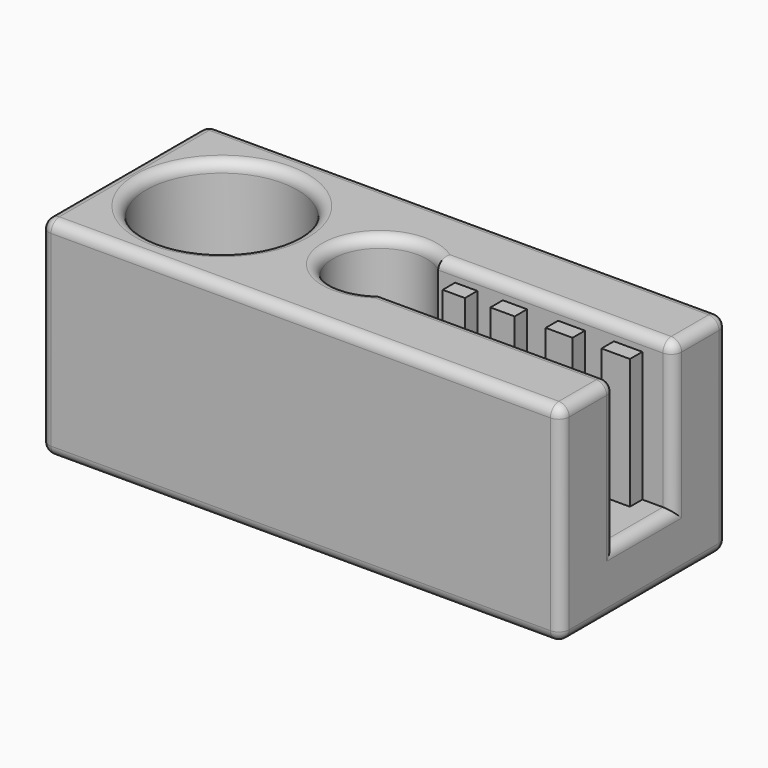
from build123d import *

# Parameters (mm, degrees)
F0_W           = 25.4
F0_H           = 10.16
F1_DEPTH       = 10.16
F2_R           = 3.6858409811
F3_DEPTH       = 6.35
F4_R           = 2.286
F5_DEPTH       = 10.161
F6_R           = 2.032
F7_DEPTH       = 3.811
F8_W           = 1.78028786
F8_H           = 7.1321626426
F9_DEPTH       = 12.7
F10_W          = 1.08565134
F10_H          = 0.7570284122
F10_W_2        = 1.1861119419
F10_W_3        = 1.3122945093
F10_W_4        = 1.3880031183
F11_DEPTH      = 6.35
F12_T1_DEPTH   = 9.144
F12_T3_DEPTH   = 2.28371214
F12_T5_DEPTH   = 6.6241626426
F12_T7_DEPTH   = 3.5605757201
F12_T9_DEPTH   = 2.28371214
F12_T11_DEPTH  = 9.144
F12_T13_DEPTH  = 24.384
F12_T15_DEPTH  = 12.2405523365
F12_S19_W      = 0.508
F12_S19_H      = 0.508
F12_T20_DEPTH  = 0.508
F12_S25_W      = 0.508
F12_S25_H      = 0.508
F12_T26_DEPTH  = 0.508
F12_S31_W      = 0.508
F12_S31_H      = 0.508
F12_T32_DEPTH  = 0.508
F12_S37_W      = 0.508
F12_S37_H      = 0.508
F12_T38_DEPTH  = 0.508
F12_S43_W      = 0.508
F12_S43_H      = 0.508
F12_T44_DEPTH  = 0.508
F12_S49_W      = 0.508
F12_S49_H      = 0.508
F12_T50_DEPTH  = 0.508
F12_S55_W      = 0.508
F12_S55_H      = 0.508
F12_T56_DEPTH  = 0.508
F12_S61_W      = 0.508
F12_S61_H      = 0.508
F12_T62_DEPTH  = 0.508
F12_S67_W      = 0.508
F12_S67_H      = 0.508
F12_T68_DEPTH  = 0.508
F12_S73_W      = 0.508
F12_S73_H      = 0.508
F12_T74_DEPTH  = 0.508
F12_T80_ANGLE  = 321.5743152005
F12_T86_ANGLE  = 82.9839978372
F12_T93_ANGLE  = 82.9839978372
F12_T99_ANGLE  = 82.9839978372
F12_T105_ANGLE = 82.9839978372
F12_T111_ANGLE = 82.9839978372
F12_T117_ANGLE = 82.9839978372
F12_T129_DEPTH = 7.8941626426
F12_T133_DEPTH = 4.8305757201
F12_T140_DEPTH = 4.8305757201
F12_T144_DEPTH = 7.8941626426


# Not quite as in the source:
# - a fillet or chamfer that OpenCascade refuses, or shapes differently, is made with other operations: its cross-section is extruded or revolved along the edge and cut away or added


with BuildPart() as f1:
    # F0 (on Front) → F1 (new body)
    with BuildSketch(Plane.XZ):
        with Locations((0.2125576138, 0.3190716813)):
            Rectangle(F0_W, F0_H)
    extrude(amount=F1_DEPTH)

    # F2 (on face) → F3 (cut)
    with BuildSketch(Plane.XY.offset(5.3990716813)):
        with Locations((-7.7062794007, -5.08)):
            Circle(F2_R)
    extrude(amount=-F3_DEPTH, mode=Mode.SUBTRACT)

    # F4 (on face) → F5 (cut, through all)
    with BuildSketch(Plane.XY.offset(5.3990716813)):
        with Locations((0, -5.08)):
            Circle(F4_R)
    extrude(amount=-F5_DEPTH, mode=Mode.SUBTRACT)

    # F6 (on face) → F7 (cut, through all)
    with BuildSketch(Plane.XY.offset(-0.9509283187)):
        with Locations((-7.7062794007, -5.08)):
            Circle(F6_R)
    extrude(amount=-F7_DEPTH, mode=Mode.SUBTRACT)

    # F8 (on face) → F9 (cut)
    with BuildSketch(Plane.YZ.offset(12.9125576138)):
        with Locations((-5.97014393, 1.83299036)):
            Rectangle(F8_W, F8_H)
        with Locations((-4.18985607, 1.83299036)):
            Rectangle(F8_W, F8_H)
    extrude(amount=-F9_DEPTH, mode=Mode.SUBTRACT)

    # F10 (on face) → F11 (join)
    with BuildSketch(Plane.XY.offset(-1.7330909614)):
        with Locations((2.8024074854, -3.6782263461)):
            Rectangle(F10_W, F10_H)
        with Locations((5.1806154661, -3.6782263461)):
            Rectangle(F10_W_2, F10_H)
        with Locations((7.9440039117, -3.6782263461)):
            Rectangle(F10_W_3, F10_H)
        with Locations((10.7073918916, -3.6782263461)):
            Rectangle(F10_W_4, F10_H)
        with Locations((2.8024074854, -6.4817736539)):
            Rectangle(F10_W, F10_H)
        with Locations((5.1806154661, -6.4817736539)):
            Rectangle(F10_W_2, F10_H)
        with Locations((7.9440039117, -6.4817736539)):
            Rectangle(F10_W_3, F10_H)
        with Locations((10.7073918916, -6.4817736539)):
            Rectangle(F10_W_4, F10_H)
    extrude(amount=F11_DEPTH)

    # F12: fillet of radius 0.508 on 25 edges, made by hand

    # F12_s2 → F12_t1 (cut)
    with BuildSketch(Plane.XY.offset(-4.2529283187)):
        with BuildLine():
            ThreePointArc((12.4045576138, 0), (12.7637678587, -0.1487897552), (12.9125576138, -0.508))
            Line((12.9125576138, -0.508), (12.9125576138, 0))
            Line((12.9125576138, 0), (12.4045576138, 0))
        make_face()
        with BuildLine():
            ThreePointArc((12.4045576138, -10.16), (12.7637678587, -10.0112102448), (12.9125576138, -9.652))
            Line((12.9125576138, -9.652), (12.9125576138, -10.16))
            Line((12.9125576138, -10.16), (12.4045576138, -10.16))
        make_face()
        with BuildLine():
            ThreePointArc((-11.9794423862, 0), (-12.338652631, -0.1487897552), (-12.4874423862, -0.508))
            Line((-12.4874423862, -0.508), (-12.4874423862, 0))
            Line((-12.4874423862, 0), (-11.9794423862, 0))
        make_face()
        with BuildLine():
            ThreePointArc((-12.4874423862, -9.652), (-12.338652631, -10.0112102448), (-11.9794423862, -10.16))
            Line((-11.9794423862, -10.16), (-12.4874423862, -10.16))
            Line((-12.4874423862, -10.16), (-12.4874423862, -9.652))
        make_face()
    extrude(amount=F12_T1_DEPTH, mode=Mode.SUBTRACT)

    # F12_s4 → F12_t3 (cut)
    with BuildSketch(Plane.XZ.offset(0.508)):
        with BuildLine():
            ThreePointArc((12.4045576138, 5.3990716813), (12.7637678587, 5.2502819261), (12.9125576138, 4.8910716813))
            Line((12.9125576138, 4.8910716813), (12.9125576138, 5.3990716813))
            Line((12.9125576138, 5.3990716813), (12.4045576138, 5.3990716813))
        make_face()
    extrude(amount=F12_T3_DEPTH, mode=Mode.SUBTRACT)

    # F12_s6 → F12_t5 (cut)
    with BuildSketch(Plane.XY.offset(-1.7330909614)):
        with BuildLine():
            ThreePointArc((12.9125576138, -2.79171214), (12.7637678587, -3.1509223848), (12.4045576138, -3.29971214))
            Line((12.4045576138, -3.29971214), (12.9125576138, -3.29971214))
            Line((12.9125576138, -3.29971214), (12.9125576138, -2.79171214))
        make_face()
        with BuildLine():
            ThreePointArc((12.9125576138, -7.36828786), (12.7637678587, -7.0090776152), (12.4045576138, -6.86028786))
            Line((12.4045576138, -6.86028786), (12.9125576138, -6.86028786))
            Line((12.9125576138, -6.86028786), (12.9125576138, -7.36828786))
        make_face()
    extrude(amount=F12_T5_DEPTH, mode=Mode.SUBTRACT)

    # F12_s8 → F12_t7 (cut)
    with BuildSketch(Plane.XZ.offset(3.29971214)):
        with BuildLine():
            ThreePointArc((12.9125576138, -2.2410909614), (12.7637678587, -1.8818807165), (12.4045576138, -1.7330909614))
            Line((12.4045576138, -1.7330909614), (12.9125576138, -1.7330909614))
            Line((12.9125576138, -1.7330909614), (12.9125576138, -2.2410909614))
        make_face()
    extrude(amount=F12_T7_DEPTH, mode=Mode.SUBTRACT)

    # F12_s10 → F12_t9 (cut)
    with BuildSketch(Plane.XZ.offset(7.36828786)):
        with BuildLine():
            ThreePointArc((12.4045576138, 5.3990716813), (12.7637678587, 5.2502819261), (12.9125576138, 4.8910716813))
            Line((12.9125576138, 4.8910716813), (12.9125576138, 5.3990716813))
            Line((12.9125576138, 5.3990716813), (12.4045576138, 5.3990716813))
        make_face()
    extrude(amount=F12_T9_DEPTH, mode=Mode.SUBTRACT)

    # F12_s12 → F12_t11 (cut)
    with BuildSketch(Plane.XZ.offset(0.508)):
        with BuildLine():
            ThreePointArc((12.9125576138, -4.2529283187), (12.7637678587, -4.6121385636), (12.4045576138, -4.7609283187))
            Line((12.4045576138, -4.7609283187), (12.9125576138, -4.7609283187))
            Line((12.9125576138, -4.7609283187), (12.9125576138, -4.2529283187))
        make_face()
        with BuildLine():
            ThreePointArc((-12.4874423862, -4.2529283187), (-12.338652631, -4.6121385636), (-11.9794423862, -4.7609283187))
            Line((-11.9794423862, -4.7609283187), (-12.4874423862, -4.7609283187))
            Line((-12.4874423862, -4.7609283187), (-12.4874423862, -4.2529283187))
        make_face()
        with BuildLine():
            ThreePointArc((-11.9794423862, 5.3990716813), (-12.338652631, 5.2502819261), (-12.4874423862, 4.8910716813))
            Line((-12.4874423862, 4.8910716813), (-12.4874423862, 5.3990716813))
            Line((-12.4874423862, 5.3990716813), (-11.9794423862, 5.3990716813))
        make_face()
    extrude(amount=F12_T11_DEPTH, mode=Mode.SUBTRACT)

    # F12_s14 → F12_t13 (cut)
    with BuildSketch(Plane.YZ.offset(-11.9794423862)):
        with BuildLine():
            ThreePointArc((-0.508, 5.3990716813), (-0.1487897552, 5.2502819261), (0, 4.8910716813))
            Line((0, 4.8910716813), (0, 5.3990716813))
            Line((0, 5.3990716813), (-0.508, 5.3990716813))
        make_face()
        with BuildLine():
            ThreePointArc((-9.652, 5.3990716813), (-10.0112102448, 5.2502819261), (-10.16, 4.8910716813))
            Line((-10.16, 4.8910716813), (-10.16, 5.3990716813))
            Line((-10.16, 5.3990716813), (-9.652, 5.3990716813))
        make_face()
        with BuildLine():
            ThreePointArc((0, -4.2529283187), (-0.1487897552, -4.6121385636), (-0.508, -4.7609283187))
            Line((-0.508, -4.7609283187), (0, -4.7609283187))
            Line((0, -4.7609283187), (0, -4.2529283187))
        make_face()
        with BuildLine():
            ThreePointArc((-10.16, -4.2529283187), (-10.0112102448, -4.6121385636), (-9.652, -4.7609283187))
            Line((-9.652, -4.7609283187), (-10.16, -4.7609283187))
            Line((-10.16, -4.7609283187), (-10.16, -4.2529283187))
        make_face()
    extrude(amount=F12_T13_DEPTH, mode=Mode.SUBTRACT)

    # F12_s16 → F12_t15 (cut)
    with BuildSketch(Plane.YZ.offset(0.1640052773)):
        with BuildLine():
            ThreePointArc((-7.36828786, 5.3990716813), (-7.0090776152, 5.2502819261), (-6.86028786, 4.8910716813))
            Line((-6.86028786, 4.8910716813), (-6.86028786, 5.3990716813))
            Line((-6.86028786, 5.3990716813), (-7.36828786, 5.3990716813))
        make_face()
        with BuildLine():
            ThreePointArc((-2.79171214, 5.3990716813), (-3.1509223848, 5.2502819261), (-3.29971214, 4.8910716813))
            Line((-3.29971214, 4.8910716813), (-3.29971214, 5.3990716813))
            Line((-3.29971214, 5.3990716813), (-2.79171214, 5.3990716813))
        make_face()
    extrude(amount=F12_T15_DEPTH, mode=Mode.SUBTRACT)


with BuildPart() as f12_tool18:
    # F12_s19 → F12_t20 (new body)
    with BuildSketch(Plane.XZ.offset(0.508)):
        with Locations((12.6585576138, -4.5069283187)):
            Rectangle(F12_S19_W, F12_S19_H)
    extrude(amount=-F12_T20_DEPTH)

    # F12_s21 → F12_t22 (revolve, cut)
    with BuildSketch(Plane(origin=(12.4045576138, -0.508, -4.2529283187), x_dir=(-0.7071067812, 0, 0.7071067812), z_dir=(-0.7071067812, 0, -0.7071067812))):
        with BuildLine():
            ThreePointArc((0, -0.508), (0.508, 0), (0, 0.508))
            Line((0, 0.508), (0, -0.508))
        make_face()
    revolve(axis=Axis((12.4045576138, -0.508, -4.2529283187), (0, 1, 0)), mode=Mode.SUBTRACT)


with BuildPart() as f1_1:
    add(f1.part)

    # F12_t17: cut F12_tool18
    add(f12_tool18.part, mode=Mode.SUBTRACT)


with BuildPart() as f12_tool24:
    # F12_s25 → F12_t26 (new body)
    with BuildSketch(Plane.XY.offset(4.8910716813)):
        with Locations((12.6585576138, -0.254)):
            Rectangle(F12_S25_W, F12_S25_H)
    extrude(amount=F12_T26_DEPTH)

    # F12_s27 → F12_t28 (revolve, cut)
    with BuildSketch(Plane(origin=(12.4045576138, -0.508, 4.8910716813), x_dir=(-0.7071067812, -0.7071067812, 0), z_dir=(-0.7071067812, 0.7071067812, 0))):
        with BuildLine():
            ThreePointArc((0, -0.508), (0.508, 0), (0, 0.508))
            Line((0, 0.508), (0, -0.508))
        make_face()
    revolve(axis=Axis((12.4045576138, -0.508, 4.8910716813), (0, 0, 1)), mode=Mode.SUBTRACT)


with BuildPart() as f1_2:
    add(f1_1.part)

    # F12_t23: cut F12_tool24
    add(f12_tool24.part, mode=Mode.SUBTRACT)


with BuildPart() as f12_tool30:
    # F12_s31 → F12_t32 (new body)
    with BuildSketch(Plane.XY.offset(4.8910716813)):
        with Locations((12.6585576138, -3.04571214)):
            Rectangle(F12_S31_W, F12_S31_H)
    extrude(amount=F12_T32_DEPTH)

    # F12_s33 → F12_t34 (revolve, cut)
    with BuildSketch(Plane(origin=(12.4045576138, -2.79171214, 4.8910716813), x_dir=(-0.7071067812, 0.7071067812, 0), z_dir=(0.7071067812, 0.7071067812, 0))):
        with BuildLine():
            ThreePointArc((0, -0.508), (0.508, 0), (0, 0.508))
            Line((0, 0.508), (0, -0.508))
        make_face()
    revolve(axis=Axis((12.4045576138, -2.79171214, 4.8910716813), (0, 0, 1)), mode=Mode.SUBTRACT)


with BuildPart() as f1_3:
    add(f1_2.part)

    # F12_t29: cut F12_tool30
    add(f12_tool30.part, mode=Mode.SUBTRACT)


with BuildPart() as f12_tool36:
    # F12_s37 → F12_t38 (new body)
    with BuildSketch(Plane.XY.offset(4.8910716813)):
        with Locations((12.6585576138, -7.11428786)):
            Rectangle(F12_S37_W, F12_S37_H)
    extrude(amount=F12_T38_DEPTH)

    # F12_s39 → F12_t40 (revolve, cut)
    with BuildSketch(Plane(origin=(12.4045576138, -7.36828786, 4.8910716813), x_dir=(-0.7071067812, -0.7071067812, 0), z_dir=(-0.7071067812, 0.7071067812, 0))):
        with BuildLine():
            ThreePointArc((0, -0.508), (0.508, 0), (0, 0.508))
            Line((0, 0.508), (0, -0.508))
        make_face()
    revolve(axis=Axis((12.4045576138, -7.36828786, 4.8910716813), (0, 0, 1)), mode=Mode.SUBTRACT)


with BuildPart() as f1_4:
    add(f1_3.part)

    # F12_t35: cut F12_tool36
    add(f12_tool36.part, mode=Mode.SUBTRACT)


with BuildPart() as f12_tool42:
    # F12_s43 → F12_t44 (new body)
    with BuildSketch(Plane.XY.offset(4.8910716813)):
        with Locations((12.6585576138, -9.906)):
            Rectangle(F12_S43_W, F12_S43_H)
    extrude(amount=F12_T44_DEPTH)

    # F12_s45 → F12_t46 (revolve, cut)
    with BuildSketch(Plane(origin=(12.4045576138, -9.652, 4.8910716813), x_dir=(-0.7071067812, 0.7071067812, 0), z_dir=(0.7071067812, 0.7071067812, 0))):
        with BuildLine():
            ThreePointArc((0, -0.508), (0.508, 0), (0, 0.508))
            Line((0, 0.508), (0, -0.508))
        make_face()
    revolve(axis=Axis((12.4045576138, -9.652, 4.8910716813), (0, 0, 1)), mode=Mode.SUBTRACT)


with BuildPart() as f1_5:
    add(f1_4.part)

    # F12_t41: cut F12_tool42
    add(f12_tool42.part, mode=Mode.SUBTRACT)


with BuildPart() as f12_tool48:
    # F12_s49 → F12_t50 (new body)
    with BuildSketch(Plane.XY.offset(-4.2529283187)):
        with Locations((12.6585576138, -9.906)):
            Rectangle(F12_S49_W, F12_S49_H)
    extrude(amount=-F12_T50_DEPTH)

    # F12_s51 → F12_t52 (revolve, cut)
    with BuildSketch(Plane(origin=(12.4045576138, -9.652, -4.2529283187), x_dir=(-0.7071067812, 0.7071067812, 0), z_dir=(-0.7071067812, -0.7071067812, 0))):
        with BuildLine():
            ThreePointArc((0, -0.508), (0.508, 0), (0, 0.508))
            Line((0, 0.508), (0, -0.508))
        make_face()
    revolve(axis=Axis((12.4045576138, -9.652, -4.2529283187), (0, 0, -1)), mode=Mode.SUBTRACT)


with BuildPart() as f1_6:
    add(f1_5.part)

    # F12_t47: cut F12_tool48
    add(f12_tool48.part, mode=Mode.SUBTRACT)


with BuildPart() as f12_tool54:
    # F12_s55 → F12_t56 (new body)
    with BuildSketch(Plane.XY.offset(4.8910716813)):
        with Locations((-12.2334423862, -0.254)):
            Rectangle(F12_S55_W, F12_S55_H)
    extrude(amount=F12_T56_DEPTH)

    # F12_s57 → F12_t58 (revolve, cut)
    with BuildSketch(Plane(origin=(-11.9794423862, -0.508, 4.8910716813), x_dir=(0.7071067812, -0.7071067812, 0), z_dir=(-0.7071067812, -0.7071067812, 0))):
        with BuildLine():
            ThreePointArc((0, -0.508), (0.508, 0), (0, 0.508))
            Line((0, 0.508), (0, -0.508))
        make_face()
    revolve(axis=Axis((-11.9794423862, -0.508, 4.8910716813), (0, 0, 1)), mode=Mode.SUBTRACT)


with BuildPart() as f1_7:
    add(f1_6.part)

    # F12_t53: cut F12_tool54
    add(f12_tool54.part, mode=Mode.SUBTRACT)


with BuildPart() as f12_tool60:
    # F12_s61 → F12_t62 (new body)
    with BuildSketch(Plane.XY.offset(4.8910716813)):
        with Locations((-12.2334423862, -9.906)):
            Rectangle(F12_S61_W, F12_S61_H)
    extrude(amount=F12_T62_DEPTH)

    # F12_s63 → F12_t64 (revolve, cut)
    with BuildSketch(Plane(origin=(-11.9794423862, -9.652, 4.8910716813), x_dir=(0.7071067812, 0.7071067812, 0), z_dir=(0.7071067812, -0.7071067812, 0))):
        with BuildLine():
            ThreePointArc((0, -0.508), (0.508, 0), (0, 0.508))
            Line((0, 0.508), (0, -0.508))
        make_face()
    revolve(axis=Axis((-11.9794423862, -9.652, 4.8910716813), (0, 0, 1)), mode=Mode.SUBTRACT)


with BuildPart() as f1_8:
    add(f1_7.part)

    # F12_t59: cut F12_tool60
    add(f12_tool60.part, mode=Mode.SUBTRACT)


with BuildPart() as f12_tool66:
    # F12_s67 → F12_t68 (new body)
    with BuildSketch(Plane.XY.offset(-4.2529283187)):
        with Locations((-12.2334423862, -0.254)):
            Rectangle(F12_S67_W, F12_S67_H)
    extrude(amount=-F12_T68_DEPTH)

    # F12_s69 → F12_t70 (revolve, cut)
    with BuildSketch(Plane(origin=(-11.9794423862, -0.508, -4.2529283187), x_dir=(0.7071067812, -0.7071067812, 0), z_dir=(0.7071067812, 0.7071067812, 0))):
        with BuildLine():
            ThreePointArc((0, -0.508), (0.508, 0), (0, 0.508))
            Line((0, 0.508), (0, -0.508))
        make_face()
    revolve(axis=Axis((-11.9794423862, -0.508, -4.2529283187), (0, 0, -1)), mode=Mode.SUBTRACT)


with BuildPart() as f1_9:
    add(f1_8.part)

    # F12_t65: cut F12_tool66
    add(f12_tool66.part, mode=Mode.SUBTRACT)


with BuildPart() as f12_tool72:
    # F12_s73 → F12_t74 (new body)
    with BuildSketch(Plane.XY.offset(-4.2529283187)):
        with Locations((-12.2334423862, -9.906)):
            Rectangle(F12_S73_W, F12_S73_H)
    extrude(amount=-F12_T74_DEPTH)

    # F12_s75 → F12_t76 (revolve, cut)
    with BuildSketch(Plane(origin=(-11.9794423862, -9.652, -4.2529283187), x_dir=(0.7071067812, 0.7071067812, 0), z_dir=(-0.7071067812, 0.7071067812, 0))):
        with BuildLine():
            ThreePointArc((0, -0.508), (0.508, 0), (0, 0.508))
            Line((0, 0.508), (0, -0.508))
        make_face()
    revolve(axis=Axis((-11.9794423862, -9.652, -4.2529283187), (0, 0, -1)), mode=Mode.SUBTRACT)


with BuildPart() as f1_10:
    add(f1_9.part)

    # F12_t71: cut F12_tool72
    add(f12_tool72.part, mode=Mode.SUBTRACT)

    # F12_s77 → F12_t78 (revolve, cut)
    with BuildSketch(Plane.XZ.offset(5.08)):
        with BuildLine():
            ThreePointArc((-3.5124384196, 5.3990716813), (-3.8716486645, 5.2502819261), (-4.0204384196, 4.8910716813))
            Line((-4.0204384196, 4.8910716813), (-4.0204384196, 5.3990716813))
            Line((-4.0204384196, 5.3990716813), (-3.5124384196, 5.3990716813))
        make_face()
    revolve(axis=Axis((-7.7062794007, -5.08, 5.3990716813), (0, 0, 1)), mode=Mode.SUBTRACT)

    # F12_s79 → F12_t80 (revolve, cut)
    with BuildSketch(Plane(origin=(1.5786075498, -4.5298739166, 0), x_dir=(0, 0, 1), z_dir=(0.329078313, -0.9443026336, 0))):
        with BuildLine():
            ThreePointArc((5.3990716813, -1.1222821698), (5.2502819261, -0.7630719249), (4.8910716813, -0.6142821698))
            Line((4.8910716813, -0.6142821698), (5.3990716813, -0.6142821698))
            Line((5.3990716813, -0.6142821698), (5.3990716813, -1.1222821698))
        make_face()
    revolve(axis=Axis((0, -5.08, 5.3990716813), (0, 0, 1)), revolution_arc=F12_T80_ANGLE, mode=Mode.SUBTRACT)

    # F12_s81 → F12_t82 (revolve, cut)
    with BuildSketch(Plane.XZ.offset(5.08)):
        with BuildLine():
            ThreePointArc((-5.1662794007, -0.9509283187), (-5.5254896456, -1.0997180739), (-5.6742794007, -1.4589283187))
            Line((-5.6742794007, -1.4589283187), (-5.6742794007, -0.9509283187))
            Line((-5.6742794007, -0.9509283187), (-5.1662794007, -0.9509283187))
        make_face()
    revolve(axis=Axis((-7.7062794007, -5.08, -0.9509283187), (0, 0, 1)), mode=Mode.SUBTRACT)


with BuildPart() as f12_tool84:
    # F12_s85 → F12_t86 (revolve)
    with BuildSketch(Plane(origin=(-0.61585817, -0.0757924774, 0), x_dir=(0, 0, 1), z_dir=(-0.992512076, -0.1221465473, 0))):
        with BuildLine():
            ThreePointArc((-2.2410909614, -7.327961346), (-1.8818807165, -7.4767511012), (-1.7330909614, -7.835961346))
            Line((-1.7330909614, -7.835961346), (-1.7330909614, -7.327961346))
            Line((-1.7330909614, -7.327961346), (-2.2410909614, -7.327961346))
        make_face()
    revolve(axis=Axis((0, -5.08, -1.7330909614), (0, 0, 1)), revolution_arc=F12_T86_ANGLE)

    split(bisect_by=Plane.XZ.offset(6.86028786), keep=Keep.BOTTOM)

    split(bisect_by=Plane.YZ.offset(2.2595818155), keep=Keep.BOTTOM)

    split(bisect_by=Plane.XZ.offset(6.1032594478), keep=Keep.TOP)


with BuildPart() as f1_11:
    add(f1_10.part)

    # F12_t83: cut F12_tool84
    add(f12_tool84.part, mode=Mode.SUBTRACT)


with BuildPart() as f12_tool91:
    # F12_s92 → F12_t93 (revolve)
    with BuildSketch(Plane(origin=(-0.61585817, -0.0757924774, 0), x_dir=(0, 0, 1), z_dir=(-0.992512076, -0.1221465473, 0))):
        with BuildLine():
            ThreePointArc((-2.2410909614, -7.327961346), (-1.8818807165, -7.4767511012), (-1.7330909614, -7.835961346))
            Line((-1.7330909614, -7.835961346), (-1.7330909614, -7.327961346))
            Line((-1.7330909614, -7.327961346), (-2.2410909614, -7.327961346))
        make_face()
    revolve(axis=Axis((0, -5.08, -1.7330909614), (0, 0, 1)), revolution_arc=F12_T93_ANGLE)

    split(bisect_by=Plane.YZ.offset(2.2595818155), keep=Keep.BOTTOM)

    split(bisect_by=Plane.XZ.offset(6.1032594478), keep=Keep.BOTTOM)


with BuildPart() as f1_12:
    add(f1_11.part)

    # F12_t90: cut F12_tool91
    add(f12_tool91.part, mode=Mode.SUBTRACT)


with BuildPart() as f12_tool97:
    # F12_s98 → F12_t99 (revolve)
    with BuildSketch(Plane(origin=(-0.61585817, -0.0757924774, 0), x_dir=(0, 0, 1), z_dir=(-0.992512076, -0.1221465473, 0))):
        with BuildLine():
            ThreePointArc((-2.2410909614, -7.327961346), (-1.8818807165, -7.4767511012), (-1.7330909614, -7.835961346))
            Line((-1.7330909614, -7.835961346), (-1.7330909614, -7.327961346))
            Line((-1.7330909614, -7.327961346), (-2.2410909614, -7.327961346))
        make_face()
    revolve(axis=Axis((0, -5.08, -1.7330909614), (0, 0, 1)), revolution_arc=F12_T99_ANGLE)

    split(bisect_by=Plane.YZ.offset(2.2595818155), keep=Keep.TOP)

    split(bisect_by=Plane.XZ.offset(6.1032594478), keep=Keep.BOTTOM)


with BuildPart() as f1_13:
    add(f1_12.part)

    # F12_t96: cut F12_tool97
    add(f12_tool97.part, mode=Mode.SUBTRACT)


with BuildPart() as f12_tool103:
    # F12_s104 → F12_t105 (revolve)
    with BuildSketch(Plane.XZ.offset(5.08)):
        with BuildLine():
            ThreePointArc((2.286, -2.2410909614), (2.4347897552, -1.8818807165), (2.794, -1.7330909614))
            Line((2.794, -1.7330909614), (2.286, -1.7330909614))
            Line((2.286, -1.7330909614), (2.286, -2.2410909614))
        make_face()
    revolve(axis=Axis((0, -5.08, -1.7330909614), (0, 0, 1)), revolution_arc=F12_T105_ANGLE)

    split(bisect_by=Plane.XZ.offset(4.0567405522), keep=Keep.TOP)

    split(bisect_by=Plane.YZ.offset(2.2595818155), keep=Keep.TOP)


with BuildPart() as f1_14:
    add(f1_13.part)

    # F12_t102: cut F12_tool103
    add(f12_tool103.part, mode=Mode.SUBTRACT)


with BuildPart() as f12_tool109:
    # F12_s110 → F12_t111 (revolve)
    with BuildSketch(Plane.XZ.offset(5.08)):
        with BuildLine():
            ThreePointArc((2.286, -2.2410909614), (2.4347897552, -1.8818807165), (2.794, -1.7330909614))
            Line((2.794, -1.7330909614), (2.286, -1.7330909614))
            Line((2.286, -1.7330909614), (2.286, -2.2410909614))
        make_face()
    revolve(axis=Axis((0, -5.08, -1.7330909614), (0, 0, 1)), revolution_arc=F12_T111_ANGLE)

    split(bisect_by=Plane.XZ.offset(4.0567405522), keep=Keep.TOP)

    split(bisect_by=Plane.YZ.offset(2.2595818155), keep=Keep.BOTTOM)


with BuildPart() as f1_15:
    add(f1_14.part)

    # F12_t108: cut F12_tool109
    add(f12_tool109.part, mode=Mode.SUBTRACT)


with BuildPart() as f12_tool115:
    # F12_s116 → F12_t117 (revolve)
    with BuildSketch(Plane.XZ.offset(5.08)):
        with BuildLine():
            ThreePointArc((2.286, -2.2410909614), (2.4347897552, -1.8818807165), (2.794, -1.7330909614))
            Line((2.794, -1.7330909614), (2.286, -1.7330909614))
            Line((2.286, -1.7330909614), (2.286, -2.2410909614))
        make_face()
    revolve(axis=Axis((0, -5.08, -1.7330909614), (0, 0, 1)), revolution_arc=F12_T117_ANGLE)

    split(bisect_by=Plane.XZ.offset(3.29971214), keep=Keep.TOP)

    split(bisect_by=Plane.XZ.offset(4.0567405522), keep=Keep.BOTTOM)

    split(bisect_by=Plane.YZ.offset(2.2595818155), keep=Keep.BOTTOM)


with BuildPart() as f1_16:
    add(f1_15.part)

    # F12_t114: cut F12_tool115
    add(f12_tool115.part, mode=Mode.SUBTRACT)

    # F12_s121 → F12_t122 (revolve, cut)
    with BuildSketch(Plane.XZ.offset(5.08)):
        with BuildLine():
            ThreePointArc((2.286, -4.2529283187), (2.4347897552, -4.6121385636), (2.794, -4.7609283187))
            Line((2.794, -4.7609283187), (2.286, -4.7609283187))
            Line((2.286, -4.7609283187), (2.286, -4.2529283187))
        make_face()
    revolve(axis=Axis((0, -5.08, -4.7609283187), (0, 0, 1)), mode=Mode.SUBTRACT)

    # F12_s123 → F12_t124 (revolve, cut)
    with BuildSketch(Plane.XZ.offset(5.08)):
        with BuildLine():
            ThreePointArc((-5.1662794007, -4.7609283187), (-5.5254896456, -4.6121385636), (-5.6742794007, -4.2529283187))
            Line((-5.6742794007, -4.2529283187), (-5.6742794007, -4.7609283187))
            Line((-5.6742794007, -4.7609283187), (-5.1662794007, -4.7609283187))
        make_face()
    revolve(axis=Axis((-7.7062794007, -5.08, -4.7609283187), (0, 0, 1)), mode=Mode.SUBTRACT)


with BuildPart() as f12_tool127:
    # F12_s128 → F12_t129 (new body)
    with BuildSketch(Plane.XY.offset(-3.0030909614)):
        with BuildLine():
            ThreePointArc((12.9125576138, -2.79171214), (12.7637678587, -3.1509223848), (12.4045576138, -3.29971214))
            Line((12.4045576138, -3.29971214), (12.9125576138, -3.29971214))
            Line((12.9125576138, -3.29971214), (12.9125576138, -2.79171214))
        make_face()
    extrude(amount=F12_T129_DEPTH)

    split(bisect_by=Plane.XY.offset(-1.7330909614), keep=Keep.BOTTOM)


with BuildPart() as f12_tool131:
    # F12_s132 → F12_t133 (new body)
    with BuildSketch(Plane.XZ.offset(6.86028786)):
        with BuildLine():
            ThreePointArc((12.9125576138, -2.2410909614), (12.7637678587, -1.8818807165), (12.4045576138, -1.7330909614))
            Line((12.4045576138, -1.7330909614), (12.9125576138, -1.7330909614))
            Line((12.9125576138, -1.7330909614), (12.9125576138, -2.2410909614))
        make_face()
    extrude(amount=-F12_T133_DEPTH)

    split(bisect_by=Plane.XZ.offset(3.29971214), keep=Keep.BOTTOM)


with BuildPart() as f12_tool127_1:
    add(f12_tool127.part)

    # F12_t135: intersect F12_tool131
    add(f12_tool131.part, mode=Mode.INTERSECT)


with BuildPart() as f1_17:
    add(f1_16.part)

    # F12_t125: cut F12_tool127
    add(f12_tool127_1.part, mode=Mode.SUBTRACT)


with BuildPart() as f12_tool138:
    # F12_s139 → F12_t140 (new body)
    with BuildSketch(Plane.XZ.offset(8.13028786)):
        with BuildLine():
            ThreePointArc((12.9125576138, -2.2410909614), (12.7637678587, -1.8818807165), (12.4045576138, -1.7330909614))
            Line((12.4045576138, -1.7330909614), (12.9125576138, -1.7330909614))
            Line((12.9125576138, -1.7330909614), (12.9125576138, -2.2410909614))
        make_face()
    extrude(amount=-F12_T140_DEPTH)

    split(bisect_by=Plane.XZ.offset(6.86028786), keep=Keep.TOP)


with BuildPart() as f12_tool142:
    # F12_s143 → F12_t144 (new body)
    with BuildSketch(Plane.XY.offset(4.8910716813)):
        with BuildLine():
            ThreePointArc((12.9125576138, -7.36828786), (12.7637678587, -7.0090776152), (12.4045576138, -6.86028786))
            Line((12.4045576138, -6.86028786), (12.9125576138, -6.86028786))
            Line((12.9125576138, -6.86028786), (12.9125576138, -7.36828786))
        make_face()
    extrude(amount=-F12_T144_DEPTH)

    split(bisect_by=Plane.XY.offset(-1.7330909614), keep=Keep.BOTTOM)


with BuildPart() as f12_tool138_1:
    add(f12_tool138.part)

    # F12_t146: intersect F12_tool142
    add(f12_tool142.part, mode=Mode.INTERSECT)


with BuildPart() as f1_18:
    add(f1_17.part)

    # F12_t136: cut F12_tool138
    add(f12_tool138_1.part, mode=Mode.SUBTRACT)


solid = f1_18.part
